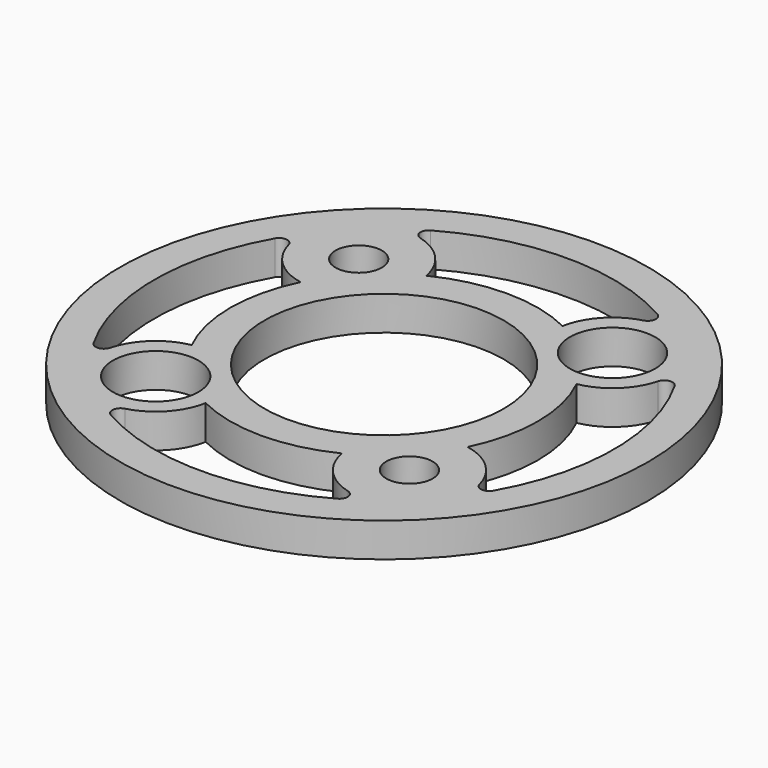
from build123d import *

# Parameters (mm, degrees)
F0_R            = 24.51608
F0_R_2          = 3.96875
F0_R_3          = 2.15265
F0_R_4          = 11.1125
F1_DEPTH        = 3.175
F3_DEPTH        = 3.175
F3_COPIES_COUNT = 4
F4_R            = 0.762


# Not quite as in the source:
# - a pattern or mirror of a feature is missing from the dataset's text; its kind, count and spacing are read off the source's solid


with BuildPart() as f1:
    # F0 (on Top) → F1 (new body)
    with BuildSketch(Plane.XY):
        Circle(F0_R)
        with Locations((-11.7865861589, -11.7865861589)):
            Circle(F0_R_2, mode=Mode.SUBTRACT)
        with Locations((11.7865861589, -11.7865861589)):
            Circle(F0_R_3, mode=Mode.SUBTRACT)
        with Locations((-11.7865861589, 11.7865861589)):
            Circle(F0_R_3, mode=Mode.SUBTRACT)
        Circle(F0_R_4, mode=Mode.SUBTRACT)
        with Locations((11.7865861589, 11.7865861589)):
            Circle(F0_R_2, mode=Mode.SUBTRACT)
    extrude(amount=F1_DEPTH)

    # F2 (on face) → F3 (cut, through all)
    with BuildSketch(Plane.XY.offset(3.175)):
        with BuildLine():
            ThreePointArc((-12.5005283394, 17.296776775), (-8.5209489043, 16.2818645023), (-6.3255746232, 12.8109235396))
            ThreePointArc((-6.3255746232, 12.8109235396), (0, 14.2875), (6.3255746232, 12.8109235396))
            ThreePointArc((6.3255746232, 12.8109235396), (8.5209489043, 16.2818645023), (12.5005283394, 17.296776775))
            ThreePointArc((12.5005283394, 17.296776775), (0, 21.34108), (-12.5005283394, 17.296776775))
        make_face()
    f3 = extrude(amount=-F3_DEPTH, mode=Mode.SUBTRACT)

    # F3_copies: F3 ×4 about axis
    f3_copies_axis = Axis((0, 0, 0), (0, 0, 1))
    for i in range(1, F3_COPIES_COUNT):
        add(f3.rotate(f3_copies_axis, i * 360 / F3_COPIES_COUNT), mode=Mode.SUBTRACT)

    # F4
    f4_edges = [f1.edges().sort_by_distance(p)[0] for p in [
        (-12.500528, 17.296777, 1.5875),
        (12.500528, 17.296777, 1.5875),
        (12.500528, -17.296777, 1.5875),
        (-12.500528, -17.296777, 1.5875),
        (17.296777, 12.500528, 1.5875),
        (17.296777, -12.500528, 1.5875),
        (-17.296777, -12.500528, 1.5875),
        (-17.296777, 12.500528, 1.5875),
    ]]
    fillet(f4_edges, radius=F4_R)


solid = f1.part
